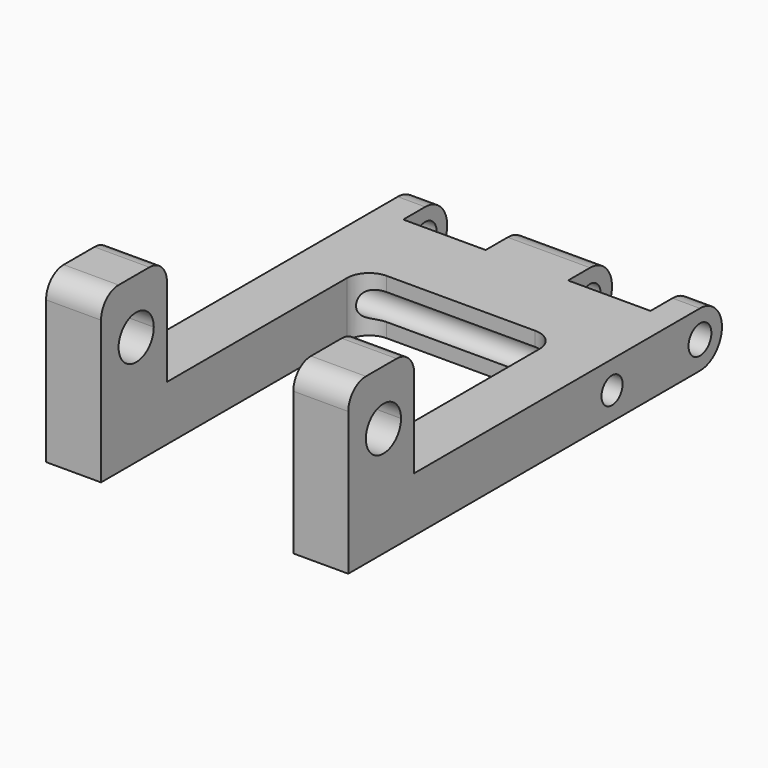
from build123d import *

# Parameters (mm, degrees)
F0_W      = 12.7
F0_H      = 25.4
F1_DEPTH  = 101.6
F2_W      = 82.55
F2_H      = 25.4
F3_DEPTH  = 69.851
F4_W      = 44.45
F4_H      = 50.8
F4_H_2    = 25.4
F5_DEPTH  = 25.4
F6_R      = 5.08
F7_R      = 6.35
F7_R_2    = 3.302
F8_DEPTH  = 69.85
F9_R      = 3.302
F10_DEPTH = 69.851
F12_DEPTH = 6.35
F13_R     = 4.8460610966
F13_R_2   = 3.048
F14_DEPTH = 19.05
F15_R     = 3.048
F16_DEPTH = 69.851
F18_R     = 7.62
F19_DEPTH = 19.05
F20_R     = 7.62
F21_DEPTH = 19.05


# Not quite as in the source:
# - two fillets or chamfers of one size are made in one step
# - a feature names something its author has since deleted; it is built from what else it names


with BuildPart() as f1:
    # F0 (on Front) → F1 (new body)
    with BuildSketch(Plane.XZ):
        Polygon((34.925, -6.35), (34.925, 6.35), (22.225, 6.35), (-22.225, 6.35), (-34.925, 6.35), (-34.925, -6.35), align=None)
        with Locations((28.575, 19.05)):
            Rectangle(F0_W, F0_H)
        with Locations((-28.575, 19.05)):
            Rectangle(F0_W, F0_H)
    extrude(amount=F1_DEPTH)

    # F2 (on face) → F3 (cut, through all)
    with BuildSketch(Plane.YZ.offset(34.925)):
        with Locations((-41.275, 19.05)):
            Rectangle(F2_W, F2_H)
        with BuildLine():
            ThreePointArc((-86.36, 19.05), (-87.8478975516, 22.6421024484), (-91.44, 24.13))
            Line((-91.44, 24.13), (-91.44, 19.05))
            Line((-91.44, 19.05), (-96.52, 19.05))
            ThreePointArc((-96.52, 19.05), (-91.44, 13.97), (-86.36, 19.05))
        make_face()
        with BuildLine():
            Line((-91.44, 19.05), (-91.44, 24.13))
            ThreePointArc((-91.44, 24.13), (-95.0321024484, 22.6421024484), (-96.52, 19.05))
            Line((-96.52, 19.05), (-91.44, 19.05))
        make_face()
    extrude(amount=-F3_DEPTH, mode=Mode.SUBTRACT)

    # F4 (on face) → F5 (cut)
    with BuildSketch(Plane.XY.offset(6.35)):
        with Locations((0, -50.8)):
            Rectangle(F4_W, F4_H)
        with Locations((0, -88.9)):
            Rectangle(F4_W, F4_H_2)
    extrude(amount=-F5_DEPTH, mode=Mode.SUBTRACT)

    # F6
    f6_edges = [f1.edges().sort_by_distance(p)[0] for p in [
        (-28.575, -101.6, 31.75),
        (-28.575, -82.55, 31.75),
        (28.575, -101.6, 31.75),
        (28.575, -82.55, 31.75),
        (22.225, -25.4, 0),
        (-22.225, -25.4, 0),
    ]]
    fillet(f6_edges, radius=F6_R)

    # F7 (on face) → F8 (join, through all)
    with BuildSketch(Plane.YZ.offset(34.925)):
        Circle(F7_R)
        Circle(F7_R_2, mode=Mode.SUBTRACT)
    extrude(amount=-F8_DEPTH)

    # F9 (on face) → F10 (cut, through all)
    with BuildSketch(Plane.YZ.offset(34.925)):
        Circle(F9_R)
    extrude(amount=-F10_DEPTH, mode=Mode.SUBTRACT)

    # F11 (on Front) → F12 (cut, symmetric)
    with BuildSketch(Plane.XZ):
        Polygon((-9.525, -12.2059704736), (-9.525, 0), (-9.525, 12.2059704736), (-28.575, 12.2059704736), (-28.575, -12.2059704736), align=None)
        Polygon((9.525, 10.1526007056), (9.525, 0), (9.525, -10.1526007056), (28.575, -10.1526007056), (28.575, 10.1526007056), align=None)
    extrude(amount=F12_DEPTH, both=True, mode=Mode.SUBTRACT)

    # F13 (on face) → F14 (join, through all)
    with BuildSketch(Plane.YZ.offset(9.525)):
        Circle(F13_R)
        Circle(F13_R_2, mode=Mode.SUBTRACT)
    extrude(amount=-F14_DEPTH)

    # F15 (on face) → F16 (cut, through all)
    with BuildSketch(Plane.YZ.offset(34.925)):
        with Locations((-25.4, 0)):
            Circle(F15_R)
    extrude(amount=-F16_DEPTH, mode=Mode.SUBTRACT)

    # F18 (on face) → F19 (cut, through all)
    with BuildSketch(Plane.YZ.offset(9.525)):
        Circle(F18_R)
    extrude(amount=F19_DEPTH, mode=Mode.SUBTRACT)

    # F20 (on face) → F21 (cut, through all)
    with BuildSketch(Plane(origin=(-9.525, 0, 0), x_dir=(0, -1, 0), z_dir=(-1, 0, 0))):
        Circle(F20_R)
    extrude(amount=F21_DEPTH, mode=Mode.SUBTRACT)


solid = f1.part
